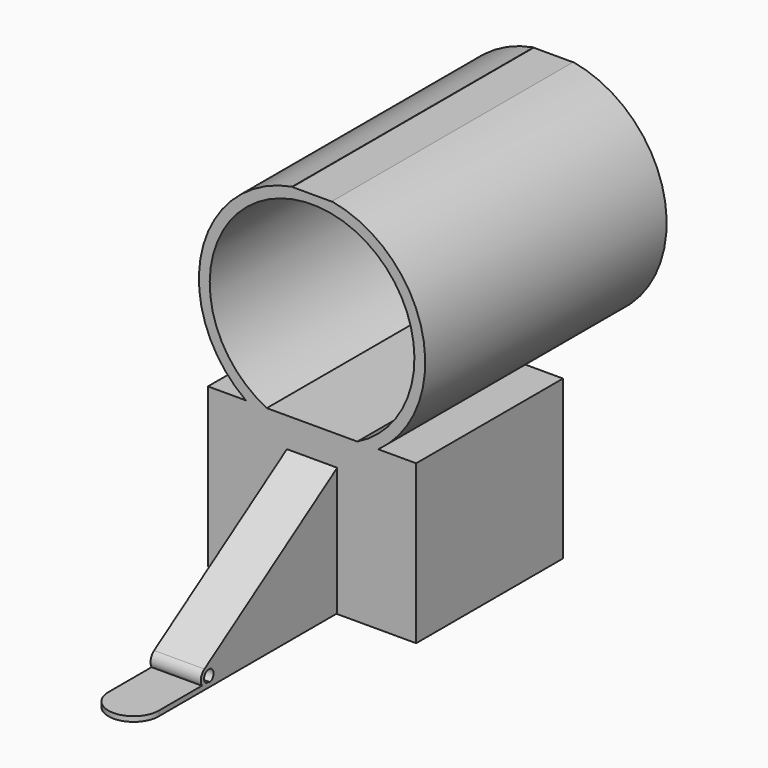
from build123d import *

# Parameters (mm, degrees)
F2_DEPTH  = 60
F3_DEPTH  = 36.5
F4_W      = 37.1
F4_H      = 32.2
F5_DEPTH  = 29.86
F7_DEPTH  = 5
F8_R      = 1.1918695684
F9_DEPTH  = 27.501
F11_DEPTH = 1


# Not quite as in the source:
# - the program builds the solid bodies; features that only make, move or delete a surface that nothing else refers to are left out


with BuildPart() as f2:
    # F0 (on Front) → F2 (new body)
    with BuildSketch(Plane.XZ):
        with BuildLine():
            Line((-9.4915752117, -20.4), (9.4915752117, -20.4))
            ThreePointArc((9.4915752117, -20.4), (11.3767265715, -19.4118544327), (13.1600721883, -18.25))
            ThreePointArc((13.1600721883, -18.25), (21.9371840047, 5.0009956954), (3.95, 22.1505643269))
            Line((3.95, 22.1505643269), (3.95, 22.1))
            Line((3.95, 22.1), (1.55, 22.1))
            Line((1.55, 22.1), (-1.55, 22.1))
            Line((-1.55, 22.1), (-3.95, 22.1))
            Line((-3.95, 22.1), (-3.95, 22.1505643269))
            ThreePointArc((-3.95, 22.1505643269), (-21.9371840047, 5.0009956954), (-13.1600721883, -18.25))
            ThreePointArc((-13.1600721883, -18.25), (-11.3767265715, -19.4118544327), (-9.4915752117, -20.4))
        make_face()
        with BuildLine():
            ThreePointArc((-9.0033327163, -18.25), (0, 20.35), (9.0033327163, -18.25))
            Line((9.0033327163, -18.25), (-3.61e-08, -18.25))
            Line((-3.61e-08, -18.25), (-9.0033327163, -18.25))
        make_face(mode=Mode.SUBTRACT)
    extrude(amount=-F2_DEPTH)

    # F0 (on Front) → F3 (join)
    with BuildSketch(Plane.XZ):
        Polygon((18.55, -20.4), (9.4915752117, -20.4), (-9.4915752117, -20.4), (-18.55, -20.4), (-18.55, -47.6), (18.55, -47.6), align=None)
        with BuildLine():
            ThreePointArc((13.1600721883, -18.25), (11.3767265715, -19.4118544327), (9.4915752117, -20.4))
            Line((9.4915752117, -20.4), (18.55, -20.4))
            Line((18.55, -20.4), (18.55, -47.6))
            Line((18.55, -47.6), (-18.55, -47.6))
            Line((-18.55, -47.6), (-18.55, -20.4))
            Line((-18.55, -20.4), (-9.4915752117, -20.4))
            ThreePointArc((-9.4915752117, -20.4), (-11.3767265715, -19.4118544327), (-13.1600721883, -18.25))
            Line((-13.1600721883, -18.25), (-15.4320283826, -18.25))
            Line((-15.4320283826, -18.25), (-20.7, -18.25))
            Line((-20.7, -18.25), (-20.7, -49.75))
            Line((-20.7, -49.75), (20.7, -49.75))
            Line((20.7, -49.75), (20.7, -18.25))
            Line((20.7, -18.25), (15.4320283826, -18.25))
            Line((15.4320283826, -18.25), (13.1600721883, -18.25))
        make_face()
    extrude(amount=-F3_DEPTH)

    # F4 (on face) → F5 (cut)
    with BuildSketch(Plane(origin=(0, 0, -49.75), x_dir=(1, 0, 0), z_dir=(0, 0, -1))):
        with Locations((0, -18.25)):
            Rectangle(F4_W, F4_H)
    extrude(amount=-F5_DEPTH, mode=Mode.SUBTRACT)


with BuildPart() as f7:
    # F6 (on Right) → F7 (new body, symmetric)
    with BuildSketch(Plane.YZ):
        with BuildLine():
            Line((-31.902618946, -49.6237426996), (0, -49.6237426996))
            Line((0, -49.6237426996), (0, -24.1335835308))
            Line((0, -24.1335835308), (-33.0056445246, -45.9554098272))
            ThreePointArc((-33.0056445246, -45.9554098272), (-33.8179081859, -48.1996481846), (-31.902618946, -49.6237426996))
        make_face()
    extrude(amount=F7_DEPTH, both=True)

    # F8 (on face) → F9 (cut, through all)
    with BuildSketch(Plane.YZ.offset(5)):
        with Locations((-31.902618946, -47.6237426996)):
            Circle(F8_R)
    extrude(amount=-F9_DEPTH, mode=Mode.SUBTRACT)

    # F10 (on face) → F11 (join)
    with BuildSketch(Plane(origin=(0, 0, -49.6237426996), x_dir=(1, 0, 0), z_dir=(0, 0, -1))):
        with BuildLine():
            Line((-5, 44.3523228168), (-5, 31.902618946))
            Line((-5, 31.902618946), (5, 31.902618946))
            Line((5, 31.902618946), (5, 44.3523228168))
            ThreePointArc((5, 44.3523228168), (0, 49.3523228168), (-5, 44.3523228168))
        make_face()
    extrude(amount=-F11_DEPTH)


solid = Compound([f2.part, f7.part])
